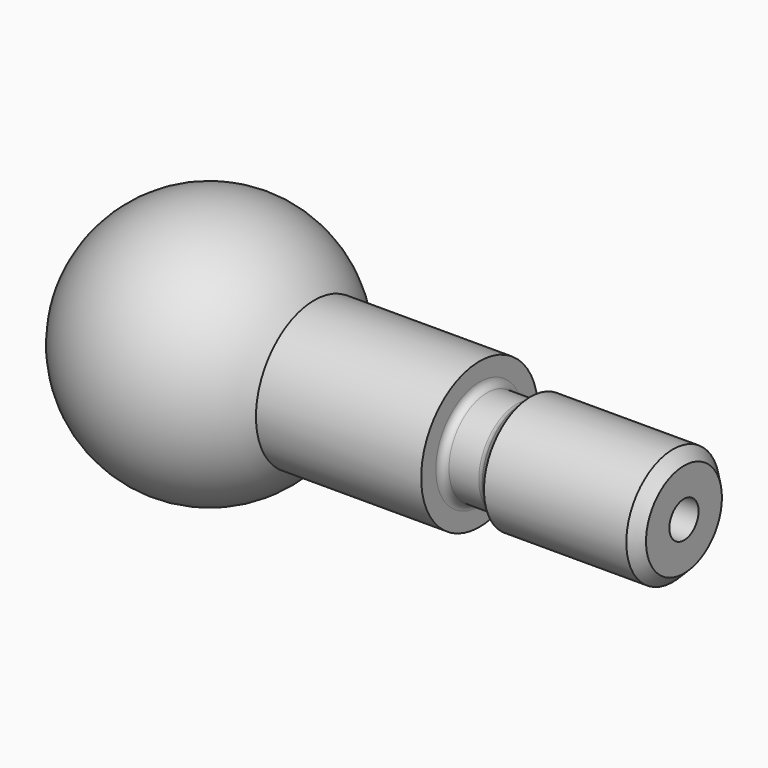
from build123d import *

# Parameters (mm, degrees)
F3_D     = 5
F3_DEPTH = 8
F3_TIP   = 1.5021515476
F4_D     = 3
F5_R     = 1
F6_SIZE  = 1.5


with BuildPart() as f1:
    # F0 (on Top) → F1 (revolve)
    with BuildSketch(Plane.XY):
        with BuildLine():
            ThreePointArc((31.8614066163, 10), (12.2595141345, 16.6969251029), (0, 0))
            Line((0, 0), (82.5, 0))
            Line((82.5, 0), (82.5, 8))
            Line((82.5, 8), (61.5, 8))
            Line((61.5, 8), (60, 6.5))
            Line((60, 6.5), (54.5, 6.5))
            Line((54.5, 6.5), (54.5, 10))
            Line((54.5, 10), (31.8614066163, 10))
        make_face()
    revolve(axis=Axis((41.25, 0, 0), (1, 0, 0)))

    # F3
    with Locations(Plane.YZ.offset(82.5)):
        with Locations((0, 0)):
            Hole(F3_D / 2, depth=F3_DEPTH)
            with Locations((0, 0, -(F3_DEPTH + F3_TIP / 2))):  # 118° drill point
                Cone(0, F3_D / 2, F3_TIP, mode=Mode.SUBTRACT)

    # F4 (through all)
    with Locations(Plane.YZ.offset(82.5)):
        with Locations((0, 0)):
            Hole(F4_D / 2)

    # F5
    f5_edges = [f1.edges().sort_by_distance(p)[0] for p in [
        (54.5, -6.5, 0),
        (60, -6.5, 0),
    ]]
    fillet(f5_edges, radius=F5_R)

    # F6
    f6_edges = [f1.edges().sort_by_distance(p)[0] for p in [
        (82.5, -8, 0),
    ]]
    chamfer(f6_edges, length=F6_SIZE)


solid = f1.part
